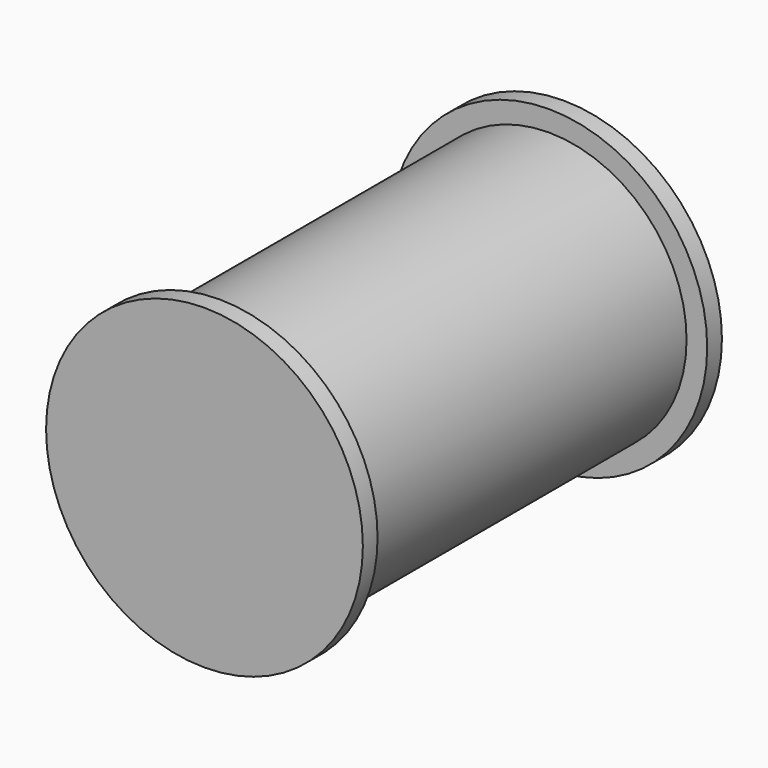
from build123d import *

# Parameters (mm, degrees)
F0_R          = 1.9020393282
F1_DEPTH      = 2.8448
F1_DEPTH_BACK = 2.8448
F2_R          = 2.1870906788
F3_DEPTH      = 0.254


# Not quite as in the source:
# - a pattern or mirror of a feature is missing from the dataset's text; its kind, count and spacing are read off the source's solid


with BuildPart() as f1:
    # F0 (on Front) → F1 (new body, two sides)
    with BuildSketch(Plane.XZ) as f1_sk:
        Circle(F0_R)
    extrude(amount=F1_DEPTH)
    extrude(f1_sk.sketch, amount=-F1_DEPTH_BACK)

    # F2 (on face) → F3 (join)
    with BuildSketch(Plane.XZ.offset(2.8448)):
        Circle(F2_R)
    f3 = extrude(amount=F3_DEPTH)

    # F3_copies: F3 across plane
    add(f3.mirror(Plane.ZX))


solid = f1.part
